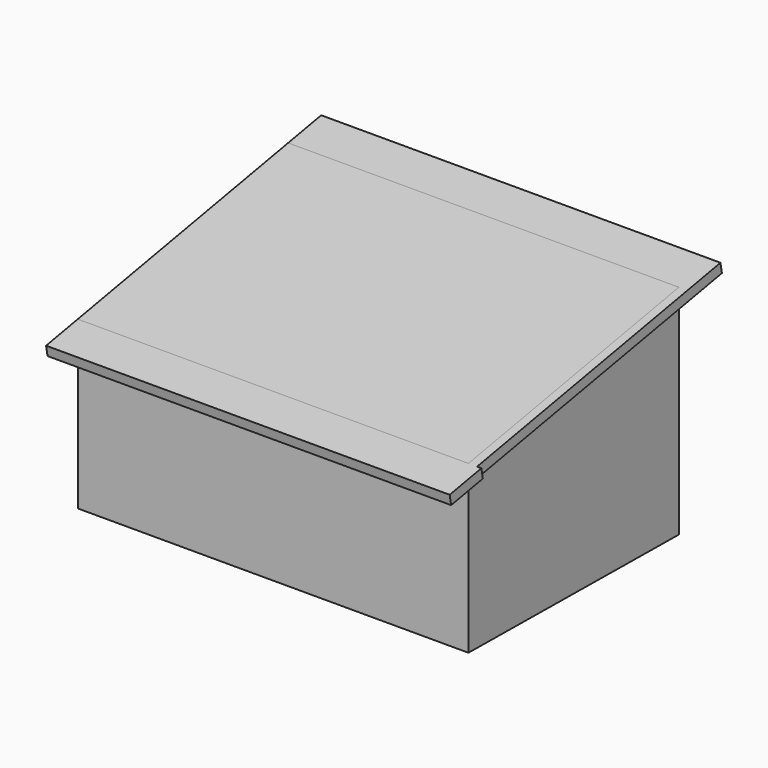
from build123d import *

# Parameters (mm, degrees)
F1_DEPTH = 138.176
F2_E3_W  = 14.2383185016
F2_E3_H  = 142.748
F3_DEPTH = 3.556
F4_E2_W  = 109.4098263908
F4_E2_H  = 141.224
F5_DEPTH = 3.556


with BuildPart() as f1:
    # F0 (on Right) → F1 (new body)
    with BuildSketch(Plane.YZ):
        Polygon((51.4731071889, 72.4924988879), (-41.5385216475, 55.4317318249), (-41.5385216475, -3.5118000333), (51.4731071889, -4.5339060016), align=None)
    extrude(amount=F1_DEPTH)

    # F2_E3 (on explicit) → F3 (join)
    with BuildSketch(Plane(origin=(0, -41.5385216475, 55.4317318249), x_dir=(0, -0.9835903566, -0.1804162143), z_dir=(0, -0.1804162143, 0.9835903566))):
        with Locations((7.1191592508, 71.374)):
            Rectangle(F2_E3_W, F2_E3_H)
    extrude(amount=-F3_DEPTH)

    # F4_E2 (on explicit) → F5 (join)
    with BuildSketch(Plane(origin=(0, 66.0759285092, 75.1710385084), x_dir=(0, -0.9835903566, -0.1804162143), z_dir=(0, -0.1804162143, 0.9835903566))):
        with Locations((54.7049131954, 70.612)):
            Rectangle(F4_E2_W, F4_E2_H)
    extrude(amount=-F5_DEPTH)


solid = f1.part
